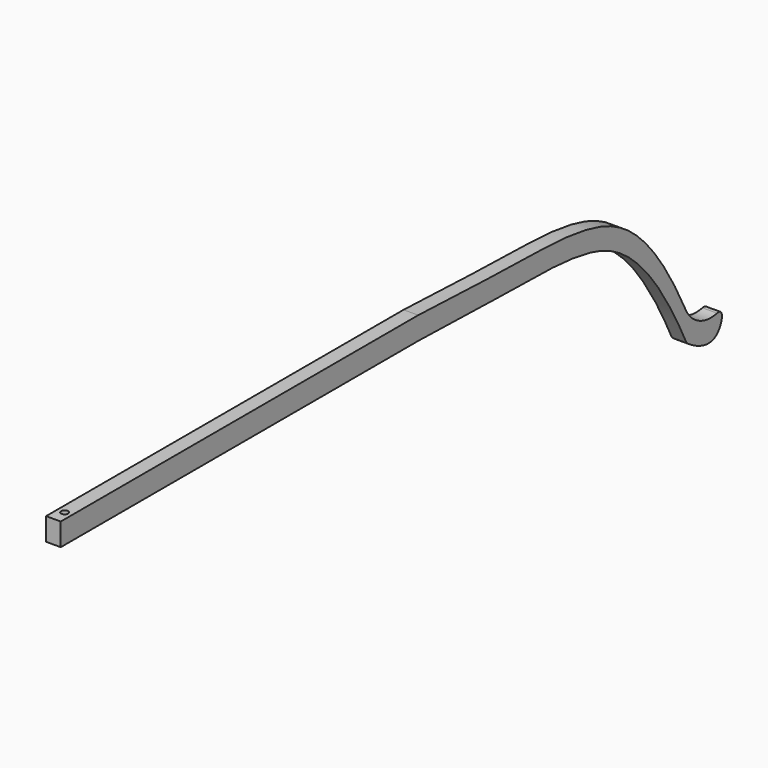
from build123d import *

# Parameters (mm, degrees)
F1_DEPTH = 2.667
F3_DEPTH = 7.62


# Not quite as in the source:
# - a feature names something its author has since deleted; it is built from what else it names


with BuildPart() as f1:
    # F0 (on Right) → F1 (new body)
    with BuildSketch(Plane.YZ):
        with BuildLine():
            Line((40.64, 2.0574), (-40.64, 2.0574))
            Line((-40.64, 2.0574), (-40.64, -2.0574))
            Line((-40.64, -2.0574), (40.64, -2.0574))
            add(Edge.make_bspline(
                [(40.64, -2.0574), (65.2363823215, -2.8826714553), (76.2322454092, -1.6712410932), (92.2423381, -7.3297932663), (101.6609776162, -27.1740333276)],
                knots=[0, 0, 0, 0, 0.5126548587, 1, 1, 1, 1], degree=3))
            add(Edge.make_bspline(
                [(108.5904209732, -25.2548671865), (108.7105657483, -25.2278232734), (110.4026487154, -24.9989116735), (108.7163421886, -31.7866160491), (102.515230767, -27.9502297874), (101.6609776162, -27.1740333276)],
                knots=[0.3182831671, 0.3182831671, 0.3182831671, 0.3182831671, 0.3383676917, 0.6233018603, 1, 1, 1, 1], degree=3))
            add(Edge.make_bspline(
                [(103.7919735763, -26.8453606559), (102.5910145162, -29.1182734519), (106.6864645495, -25.6834370678), (108.5904209732, -25.2548671865)],
                knots=[0, 0, 0, 0, 0.3182831671, 0.3182831671, 0.3182831671, 0.3182831671], degree=3))
            add(Edge.make_bspline(
                [(101.4876463788, -21.8415304228), (102.2436901965, -23.3930273167), (103.0115093513, -25.0580021652), (103.7919735763, -26.8453606559)],
                knots=[0.9590345904, 0.9590345904, 0.9590345904, 0.9590345904, 1, 1, 1, 1], degree=3))
            add(Edge.make_bspline(
                [(40.64, 2.0574), (65.0790578645, 0.8669100168), (78.5265501087, 2.3760846123), (93.2067806774, -4.8481536974), (101.4876463788, -21.8415304228)],
                knots=[0, 0, 0, 0, 0.5103449149, 0.9590345904, 0.9590345904, 0.9590345904, 0.9590345904], degree=3))
        make_face()
        with BuildLine():
            ThreePointArc((108.5904209732, -25.2548671865), (104.4454971864, -24.7832822995), (101.4876463788, -21.8415304228))
            add(Edge.make_bspline(
                [(101.4876463788, -21.8415304228), (102.2436901965, -23.3930273167), (103.0115093513, -25.0580021652), (103.7919735763, -26.8453606559)],
                knots=[0.9590345904, 0.9590345904, 0.9590345904, 0.9590345904, 1, 1, 1, 1], degree=3))
            add(Edge.make_bspline(
                [(103.7919735763, -26.8453606559), (102.5910145162, -29.1182734519), (106.6864645495, -25.6834370678), (108.5904209732, -25.2548671865)],
                knots=[0, 0, 0, 0, 0.3182831671, 0.3182831671, 0.3182831671, 0.3182831671], degree=3))
        make_face()
    extrude(amount=F1_DEPTH)

    # F2 (on face) → F3 (cut)
    with BuildSketch(Plane.XY.offset(2.0574)):
        with BuildLine():
            Line((0.6985, -38.1), (1.9685, -38.1))
            ThreePointArc((1.9685, -38.1), (1.3335, -37.465), (0.6985, -38.1))
        make_face()
        with BuildLine():
            ThreePointArc((0.6985, -38.1), (1.3335, -38.735), (1.9685, -38.1))
            Line((1.9685, -38.1), (0.6985, -38.1))
        make_face()
    extrude(amount=-F3_DEPTH, mode=Mode.SUBTRACT)


solid = f1.part
